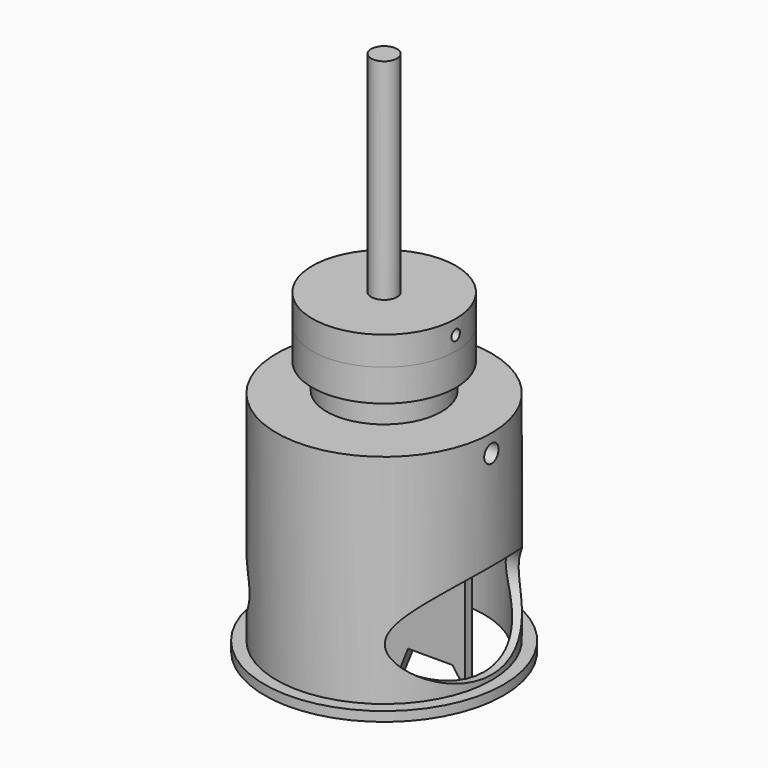
from build123d import *

# Parameters (mm, degrees)
F0_R           = 3.429
F1_DEPTH       = 50.8
F1_DEPTH_BACK  = 38.1
F3_DEPTH       = 1.143
F3_DEPTH_BACK  = 1.143
F5_R           = 28.575
F5_R_2         = 12.7
F6_DEPTH       = 9.525
F7_R           = 28.575
F7_R_2         = 26.543
F8_DEPTH       = 50.8
F9_R           = 31.75
F9_R_2         = 28.575
F10_DEPTH      = 2.54
F11_R          = 2.38125
F12_DEPTH      = 31.751
F13_R          = 12.7
F13_R_2        = 10.16
F14_DEPTH      = 10.16
F15_R          = 15.24
F15_R_2        = 3.556
F16_DEPTH      = 6.35
F17_R          = 6
F17_R_2        = 3.556
F18_DEPTH      = 8.5
F19_R          = 19.05
F19_R_2        = 14
F20_DEPTH      = 8
F25_DEPTH      = 31.751
F25_DEPTH_BACK = 31.751
F26_R          = 14
F26_R_2        = 6
F27_DEPTH      = 8
F28_R          = 19.05
F28_R_2        = 14
F29_DEPTH      = 0.5
F22_R          = 19.05
F22_R_2        = 3.429
F30_DEPTH      = 7.62
F23_R          = 1.397
F31_DEPTH      = 25.4
F32_R          = 14
F32_R_2        = 12.73
F33_DEPTH      = 0.5
F34_R          = 7.27
F34_R_2        = 6
F35_DEPTH      = 0.5


with BuildPart() as f1:
    # F0 (on Top) → F1 (new body, two sides)
    with BuildSketch(Plane.XY) as f1_sk:
        Circle(F0_R)
    extrude(amount=F1_DEPTH)
    extrude(f1_sk.sketch, amount=-F1_DEPTH_BACK)

    # F2 (on Front) → F3 (join, two sides)
    with BuildSketch(Plane.XZ) as f3_sk:
        with BuildLine():
            Line((3.429, -38.1), (-3.429, -38.1))
            add(Edge.make_bspline(
                [(-3.429, -38.1), (-5.683469061, -43.1850896463), (-12.3093663445, -43.9167752606), (-22.3240866788, -48.9271160358), (-22.429, -53.7083)],
                knots=[0, 0, 0, 0, 0.4876416588, 1, 1, 1, 1], degree=3))
            Line((-22.429, -53.7083), (-22.429, -90.0960937142))
            Line((-22.429, -90.0960937142), (-19.0627388656, -85.4583))
            Line((-19.0627388656, -85.4583), (-7.2766612284, -85.4583))
            Line((-7.2766612284, -85.4583), (0, -103.6282554269))
            Line((0, -103.6282554269), (7.2766612284, -85.4583))
            Line((7.2766612284, -85.4583), (19.0627388656, -85.4583))
            Line((19.0627388656, -85.4583), (22.429, -90.0960937142))
            Line((22.429, -90.0960937142), (22.429, -53.7083))
            add(Edge.make_bspline(
                [(3.429, -38.1), (5.683469061, -43.1850896463), (12.3093663445, -43.9167752606), (22.3240866788, -48.9271160358), (22.429, -53.7083)],
                knots=[0, 0, 0, 0, 0.4876416588, 1, 1, 1, 1], degree=3))
        make_face()
    extrude(amount=F3_DEPTH)
    extrude(f3_sk.sketch, amount=-F3_DEPTH_BACK)


with BuildPart() as f6:
    # F5 (on offset) → F6 (new body)
    with BuildSketch(Plane.XY.offset(-38.1)):
        Circle(F5_R)
        Circle(F5_R_2, mode=Mode.SUBTRACT)
    extrude(amount=F6_DEPTH)

    # F7 (on face) → F8 (join)
    with BuildSketch(Plane(origin=(0, 0, -38.1), x_dir=(1, 0, 0), z_dir=(0, 0, -1))):
        Circle(F7_R)
        Circle(F7_R_2, mode=Mode.SUBTRACT)
    extrude(amount=F8_DEPTH)

    # F9 (on face) → F10 (join)
    with BuildSketch(Plane(origin=(0, 0, -88.9), x_dir=(1, 0, 0), z_dir=(0, 0, -1))):
        Circle(F9_R)
        Circle(F9_R_2, mode=Mode.SUBTRACT)
    extrude(amount=-F10_DEPTH)

    # F11 (on Right) → F12 (cut, through all)
    with BuildSketch(Plane.YZ):
        with Locations((0, -33.3375)):
            Circle(F11_R)
    extrude(amount=F12_DEPTH, mode=Mode.SUBTRACT)

    # F24 (on Right) → F25 (cut, two sides)
    with BuildSketch(Plane.YZ) as f25_sk:
        with BuildLine():
            add(Edge.make_bspline(
                [(22.225, -72.39), (22.225, -50.3929547439), (-11.1125, -61.3914773719), (-44.45, -72.39), (-11.1125, -83.3885226281), (22.225, -94.3870452561), (22.225, -72.39)],
                knots=[0, 0, 0, 2.0943951024, 2.0943951024, 4.1887902048, 4.1887902048, 6.2831853072, 6.2831853072, 6.2831853072], degree=2, weights=[1, 0.5, 1, 0.5, 1, 0.5, 1]))
        make_face()
    extrude(amount=F25_DEPTH, mode=Mode.SUBTRACT)
    extrude(f25_sk.sketch, amount=-F25_DEPTH_BACK, mode=Mode.SUBTRACT)


with BuildPart() as f14:
    # F13 (on face) → F14 (new body)
    with BuildSketch(Plane(origin=(0, 0, -38.1), x_dir=(1, 0, 0), z_dir=(0, 0, -1))):
        Circle(F13_R)
        Circle(F13_R_2, mode=Mode.SUBTRACT)
    extrude(amount=-F14_DEPTH)

    # F15 (on face) → F16 (join)
    with BuildSketch(Plane.XY.offset(-27.94)):
        Circle(F15_R)
        Circle(F15_R_2, mode=Mode.SUBTRACT)
    extrude(amount=F16_DEPTH)

    # F17 (on face) → F18 (join)
    with BuildSketch(Plane.XY.offset(-21.59)):
        Circle(F17_R)
        Circle(F17_R_2, mode=Mode.SUBTRACT)
    extrude(amount=F18_DEPTH)

    # F34 (on face) → F35 (join)
    with BuildSketch(Plane.XY.offset(-21.59)):
        Circle(F34_R)
        Circle(F34_R_2, mode=Mode.SUBTRACT)
    extrude(amount=F35_DEPTH)


with BuildPart() as f20:
    # F19 (on face) → F20 (new body)
    with BuildSketch(Plane.XY.offset(-13.09)):
        Circle(F19_R)
        Circle(F19_R_2, mode=Mode.SUBTRACT)
    extrude(amount=-F20_DEPTH)

    # F28 (on offset) → F29 (join, through all)
    with BuildSketch(Plane.XY.offset(-12.59)):
        Circle(F28_R)
        Circle(F28_R_2, mode=Mode.SUBTRACT)
    extrude(amount=-F29_DEPTH)

    # F22 (on offset) → F30 (join)
    with BuildSketch(Plane.XY.offset(-12.59)):
        Circle(F22_R)
        Circle(F22_R_2, mode=Mode.SUBTRACT)
    extrude(amount=F30_DEPTH)

    # F23 (on Right) → F31 (cut)
    with BuildSketch(Plane.YZ):
        with Locations((0, -8.78)):
            Circle(F23_R)
    extrude(amount=F31_DEPTH, mode=Mode.SUBTRACT)

    # F32 (on face) → F33 (join)
    with BuildSketch(Plane(origin=(0, 0, -12.59), x_dir=(1, 0, 0), z_dir=(0, 0, -1))):
        Circle(F32_R)
        Circle(F32_R_2, mode=Mode.SUBTRACT)
    extrude(amount=F33_DEPTH)


with BuildPart() as f27:
    # F26 (on face) → F27 (new body)
    with BuildSketch(Plane.XY.offset(-13.09)):
        Circle(F26_R)
        Circle(F26_R_2, mode=Mode.SUBTRACT)
    extrude(amount=-F27_DEPTH)


solid = Compound([f1.part, f6.part, f14.part, f20.part, f27.part])
